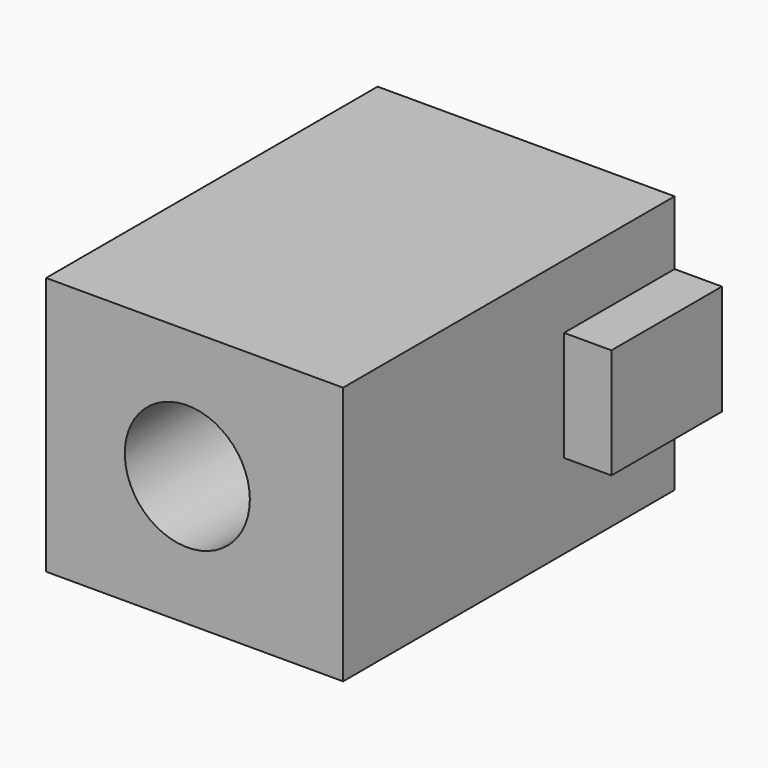
from build123d import *

# Parameters (mm, degrees)
F1_W     = 8.7014986202
F1_H     = 20.2537979931
F2_DEPTH = 25.4
F1_W_2   = 24.8446604237
F1_H_2   = 10.5319754221
F0_W     = 54.6130314469
F0_H     = 47.5477091968
F0_R     = 11.4985783996
F3_DEPTH = 50.8


with BuildPart() as f2:
    # F1 (on Front) → F2 (new body)
    with BuildSketch(Plane.XZ):
        with Locations((4.3507493101, 29.273130931)):
            Rectangle(F1_W, F1_H)
    extrude(amount=F2_DEPTH)


with BuildPart() as f2b:
    # F1 (on Front) → F2, piece 2 (new body)
    with BuildSketch(Plane.XZ):
        with Locations((-27.2152391262, -1.7826945987)):
            Rectangle(F1_W_2, F1_H_2)
    extrude(amount=F2_DEPTH)


with BuildPart() as f2c:
    # F0 (on Front) → F2, piece 3 (new body)
    with BuildSketch(Plane.XZ):
        with Locations((-27.3065157235, 27.4019930512)):
            Rectangle(F0_W, F0_H)
        with Locations((-28.6431983113, 27.4974703789)):
            Circle(F0_R, mode=Mode.SUBTRACT)
    extrude(amount=F2_DEPTH)

    # F3 (add): a face of the model
    f3_faces = [f2c.faces().sort_by_distance(p)[0] for p in [
        (-27.3065157235, -25.4, 50.4517366185),
    ]]
    extrude(f3_faces, amount=F3_DEPTH)


solid = Compound([f2.part, f2b.part, f2c.part])
